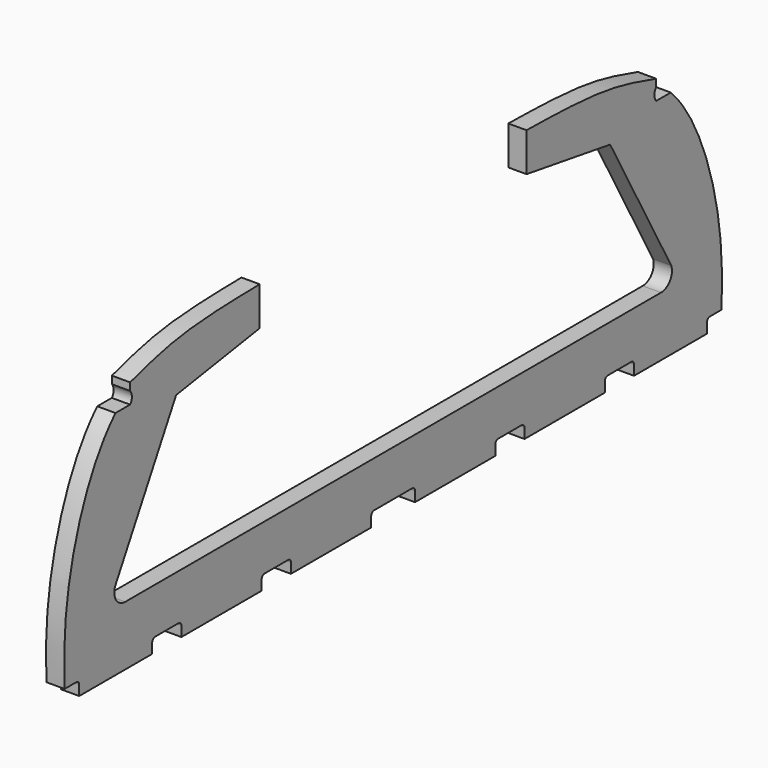
from build123d import *

# Parameters (mm, degrees)
F1_DEPTH = 25.4


with BuildPart() as f1:
    # F0 (on Right) → F1 (new body)
    with BuildSketch(Plane.YZ):
        with BuildLine():
            Line((-33.02, -94.7882861604), (0, -94.7882861604))
            Line((0, -94.7882861604), (33.02, -94.7882861604))
            ThreePointArc((33.02, -94.7882861604), (36.6121024484, -96.276183712), (38.1, -99.8682861604))
            Line((38.1, -99.8682861604), (38.1, -113.8382861604))
            Line((38.1, -113.8382861604), (177.8, -113.8382861604))
            Line((177.8, -113.8382861604), (177.8, -99.8682861604))
            ThreePointArc((177.8, -99.8682861604), (179.2878975516, -96.276183712), (182.88, -94.7882861604))
            Line((182.88, -94.7882861604), (223.52, -94.7882861604))
            ThreePointArc((223.52, -94.7882861604), (227.1121024484, -96.276183712), (228.6, -99.8682861604))
            Line((228.6, -99.8682861604), (228.6, -113.8382861604))
            Line((228.6, -113.8382861604), (368.3, -113.8382861604))
            Line((368.3, -113.8382861604), (368.3, -99.8682861604))
            ThreePointArc((368.3, -99.8682861604), (369.7878975516, -96.276183712), (373.38, -94.7882861604))
            Line((373.38, -94.7882861604), (414.02, -94.7882861604))
            ThreePointArc((414.02, -94.7882861604), (417.6121024484, -96.276183712), (419.1, -99.8682861604))
            Line((419.1, -99.8682861604), (419.1, -113.8382861604))
            Line((419.1, -113.8382861604), (546.1, -113.8382861604))
            Line((546.1, -113.8382861604), (546.1, -99.8682861604))
            ThreePointArc((546.1, -99.8682861604), (547.5878975516, -96.276183712), (551.18, -94.7882861604))
            Line((551.18, -94.7882861604), (571.5, -94.7882861604))
            add(Edge.make_bspline(
                [(571.5, -94.7882861604), (572.9916402115, -51.8796445459), (572.0651404012, 35.9396927338), (525.960624218, 164.5377278328), (483.0139090485, 207.2824090719)],
                knots=[0, 0, 0, 0, 0.455226695, 1, 1, 1, 1], degree=3))
            Line((483.0139090485, 207.2824090719), (457.6139090485, 207.2824090719))
            ThreePointArc((457.6139090485, 207.2824090719), (454.4468485925, 215.6736583026), (457.6139090485, 224.0649075333))
            Line((457.6139090485, 224.0649075333), (457.6139090485, 234.5455965156))
            add(Edge.make_bspline(
                [(457.6139090485, 234.5455965156), (430.2923400603, 242.6197356959), (367.9016901724, 260.6701177346), (280.7948912625, 262.2175910558), (232.0806728363, 263.0830109119)],
                knots=[0.0166181854, 0.0166181854, 0.0166181854, 0.0166181854, 0.4500466426, 1, 1, 1, 1], degree=3))
            Line((232.0806728363, 263.0830109119), (232.0806728363, 209.2051863447))
            Line((232.0806728363, 209.2051863447), (377.5198757648, 186.3945573568))
            Line((377.5198757648, 186.3945573568), (483.9270131228, -5.2314990347))
            ThreePointArc((483.9270131228, -5.2314990347), (481.6642820093, -22.7701705112), (465.9854230078, -30.9493104209))
            Line((465.9854230078, -30.9493104209), (0, -30.9493104209))
            Line((0, -30.9493104209), (-465.9854230078, -30.9493104209))
            ThreePointArc((-465.9854230078, -30.9493104209), (-481.6642820093, -22.7701705112), (-483.9270131228, -5.2314990347))
            Line((-483.9270131228, -5.2314990347), (-377.5198757648, 186.3945573568))
            Line((-377.5198757648, 186.3945573568), (-232.0806728363, 209.2051863447))
            Line((-232.0806728363, 209.2051863447), (-232.0806728363, 263.0830109119))
            add(Edge.make_bspline(
                [(-457.6139090485, 234.5455965156), (-430.2923400603, 242.6197356959), (-367.9016901724, 260.6701177346), (-280.7948912625, 262.2175910558), (-232.0806728363, 263.0830109119)],
                knots=[0.0166181854, 0.0166181854, 0.0166181854, 0.0166181854, 0.4500466426, 1, 1, 1, 1], degree=3))
            Line((-457.6139090485, 234.5455965156), (-457.6139090485, 224.0649075333))
            ThreePointArc((-457.6139090485, 224.0649075333), (-454.4468485925, 215.6736583026), (-457.6139090485, 207.2824090719))
            Line((-457.6139090485, 207.2824090719), (-483.0139090485, 207.2824090719))
            add(Edge.make_bspline(
                [(-571.5, -94.7882861604), (-572.9916402115, -51.8796445459), (-572.0651404012, 35.9396927338), (-525.960624218, 164.5377278328), (-483.0139090485, 207.2824090719)],
                knots=[0, 0, 0, 0, 0.455226695, 1, 1, 1, 1], degree=3))
            Line((-571.5, -94.7882861604), (-551.18, -94.7882861604))
            ThreePointArc((-551.18, -94.7882861604), (-547.5878975516, -96.276183712), (-546.1, -99.8682861604))
            Line((-546.1, -99.8682861604), (-546.1, -113.8382861604))
            Line((-546.1, -113.8382861604), (-419.1, -113.8382861604))
            Line((-419.1, -113.8382861604), (-419.1, -99.8682861604))
            ThreePointArc((-419.1, -99.8682861604), (-417.6121024484, -96.276183712), (-414.02, -94.7882861604))
            Line((-414.02, -94.7882861604), (-373.38, -94.7882861604))
            ThreePointArc((-373.38, -94.7882861604), (-369.7878975516, -96.276183712), (-368.3, -99.8682861604))
            Line((-368.3, -99.8682861604), (-368.3, -113.8382861604))
            Line((-368.3, -113.8382861604), (-228.6, -113.8382861604))
            Line((-228.6, -113.8382861604), (-228.6, -99.8682861604))
            ThreePointArc((-228.6, -99.8682861604), (-227.1121024484, -96.276183712), (-223.52, -94.7882861604))
            Line((-223.52, -94.7882861604), (-182.88, -94.7882861604))
            ThreePointArc((-182.88, -94.7882861604), (-179.2878975516, -96.276183712), (-177.8, -99.8682861604))
            Line((-177.8, -99.8682861604), (-177.8, -113.8382861604))
            Line((-177.8, -113.8382861604), (-38.1, -113.8382861604))
            Line((-38.1, -113.8382861604), (-38.1, -99.8682861604))
            ThreePointArc((-38.1, -99.8682861604), (-36.6121024484, -96.276183712), (-33.02, -94.7882861604))
        make_face()
    extrude(amount=F1_DEPTH)


solid = f1.part
